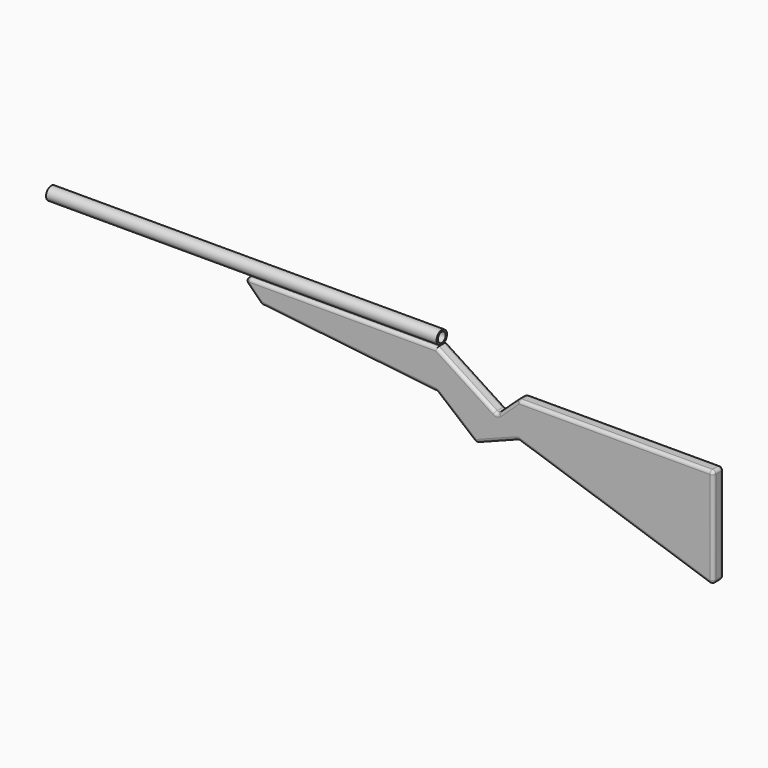
from build123d import *

# Parameters (mm, degrees)
F0_R     = 10
F1_DEPTH = 300
F2_R     = 7.5
F3_DEPTH = 300
F6_DEPTH = 10
F8_R     = 5


with BuildPart() as f1:
    # F0 (on Right) → F1 (new body)
    with BuildSketch(Plane.YZ):
        Circle(F0_R)
    extrude(amount=F1_DEPTH)

    # F2 (on face) → F3 (cut)
    with BuildSketch(Plane.YZ.offset(300)):
        Circle(F2_R)
    extrude(amount=-F3_DEPTH, mode=Mode.SUBTRACT)

    # F4: F1 across plane


with BuildPart() as f1_1:
    add(f1.part)
    add(f1.part.mirror(Plane.YZ))


with BuildPart() as f6:
    # F5 (on Front) → F6 (new body)
    with BuildSketch(Plane.XZ):
        Polygon((300, -10), (0, -10), (30, -40), (300, -70), (360, -120), (425, -95), (725, -195), (725, -95), (725, -40), (425, -40), (392.5, -70), align=None)
    extrude(amount=F6_DEPTH)

    # F7: F6 across face


with BuildPart() as f6_1:
    add(f6.part)
    add(f6.part.mirror(Plane(origin=(460.7482537362, 0, -77.3639538661), x_dir=(1, 0, 0), z_dir=(0, 1, 0))))

    # F8
    f8_edges = [f6_1.edges().sort_by_distance(p)[0] for p in [
        (15, -10, -25),
        (15, 10, -25),
        (165, 10, -55),
        (165, -10, -55),
        (30, 0, -40),
        (330, -10, -95),
        (330, 10, -95),
        (392.5, -10, -107.5),
        (392.5, 10, -107.5),
        (575, 10, -145),
        (575, -10, -145),
        (725, -10, -117.5),
        (575, -10, -40),
        (408.75, -10, -55),
        (346.25, -10, -40),
        (150, -10, -10),
        (150, 10, -10),
        (346.25, 10, -40),
        (575, 10, -40),
        (408.75, 10, -55),
        (392.5, 0, -70),
        (425, 0, -40),
        (725, 10, -117.5),
        (725, 0, -40),
        (725, 0, -195),
        (425, 0, -95),
        (360, 0, -120),
        (300, 0, -70),
        (0, 0, -10),
    ]]
    fillet(f8_edges, radius=F8_R)


solid = Compound([f1_1.part, f6_1.part])
